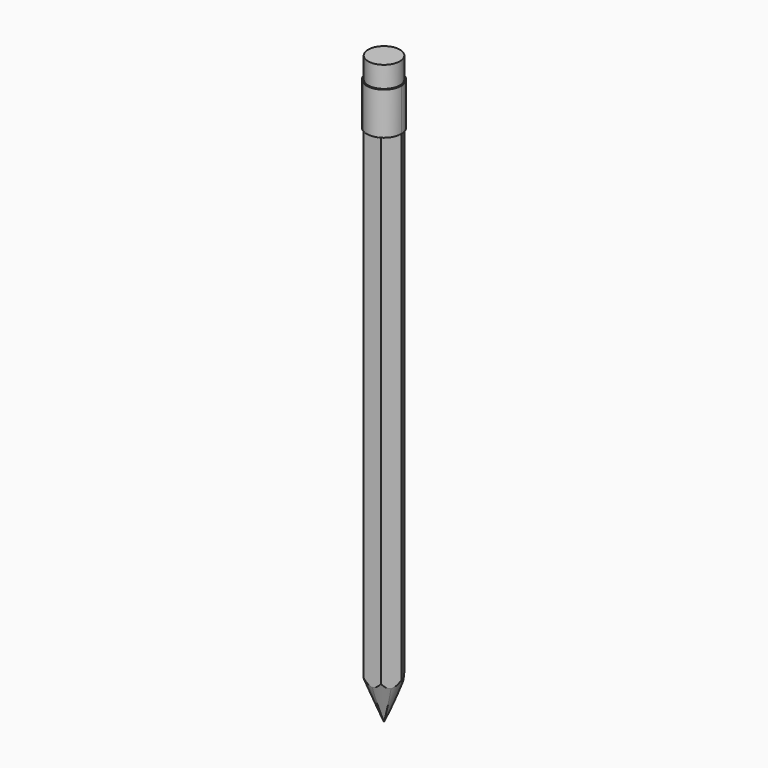
from build123d import *

# Parameters (mm, degrees)
F1_DEPTH     = 2540
F3_DEPTH     = 203.2
F4_R         = 76.1921609871
F5_DEPTH     = 101.6
F6_SIZE2     = 203.2
F6_SIZE      = 71.882
F7_T1_DEPTH  = 494.4083201135
F7_T3_DEPTH  = 494.4083201135
F7_T5_DEPTH  = 494.4083201135
F7_T7_DEPTH  = 494.4083201135
F7_T9_DEPTH  = 494.4083201135
F7_T11_DEPTH = 494.4083201135


# Not quite as in the source:
# - a fillet or chamfer that OpenCascade refuses, or shapes differently, is made with other operations: its cross-section is extruded or revolved along the edge and cut away or added


with BuildPart() as f1:
    # F0 (on Top) → F1 (new body)
    with BuildSketch(Plane.XY):
        Polygon((42.1619373396, -71.5559341018), (83.0502253935, 0.735341758), (40.8882880539, 72.2912758598), (-42.1619373396, 71.5559341018), (-83.0502253935, -0.735341758), (-40.8882880539, -72.2912758598), align=None)
    extrude(amount=F1_DEPTH)

    # F2 (on face) → F3 (join)
    with BuildSketch(Plane.XY.offset(2540)):
        with BuildLine():
            ThreePointArc((-40.8882880539, -72.2912758598), (0.735341758, -83.0502253935), (42.1619373396, -71.5559341018))
            Line((42.1619373396, -71.5559341018), (-40.8882880539, -72.2912758598))
        make_face()
        with BuildLine():
            ThreePointArc((-83.0502253935, -0.735341758), (-71.5559341018, -42.1619373396), (-40.8882880539, -72.2912758598))
            Line((-40.8882880539, -72.2912758598), (-83.0502253935, -0.735341758))
        make_face()
        with BuildLine():
            Line((-83.0502253935, -0.735341758), (-42.1619373396, 71.5559341018))
            ThreePointArc((-42.1619373396, 71.5559341018), (-72.2912758598, 40.8882880539), (-83.0502253935, -0.735341758))
        make_face()
        Polygon((42.1619373396, -71.5559341018), (83.0502253935, 0.735341758), (40.8882880539, 72.2912758598), (-42.1619373396, 71.5559341018), (-83.0502253935, -0.735341758), (-40.8882880539, -72.2912758598), align=None)
        with BuildLine():
            ThreePointArc((42.1619373396, -71.5559341018), (72.1095566371, -41.2079180135), (83.0534807543, 0))
            ThreePointArc((83.0534807543, 0), (83.0526669101, 0.3676744818), (83.0502253935, 0.735341758))
            Line((83.0502253935, 0.735341758), (42.1619373396, -71.5559341018))
        make_face()
        with BuildLine():
            Line((40.8882880539, 72.2912758598), (83.0502253935, 0.735341758))
            ThreePointArc((83.0502253935, 0.735341758), (71.5559341018, 42.1619373396), (40.8882880539, 72.2912758598))
        make_face()
        with BuildLine():
            Line((-42.1619373396, 71.5559341018), (40.8882880539, 72.2912758598))
            ThreePointArc((40.8882880539, 72.2912758598), (-0.735341758, 83.0502253935), (-42.1619373396, 71.5559341018))
        make_face()
    extrude(amount=F3_DEPTH)

    # F4 (on face) → F5 (join)
    with BuildSketch(Plane.XY.offset(2743.2)):
        Circle(F4_R)
    extrude(amount=F5_DEPTH)

    # F6
    f6_edges = [f1.edges().sort_by_distance(p)[0] for p in [
        (62.606081, -35.410296, 0),
        (61.969257, 36.513309, 0),
        (-0.636825, 71.923605, 0),
        (-62.606081, 35.410296, 0),
        (-61.969257, -36.513309, 0),
        (0.636825, -71.923605, 0),
    ]]
    f6_side = f1.faces().sort_by_distance((0, 0, 0))[0]
    chamfer(f6_edges, length=F6_SIZE, length2=F6_SIZE2, reference=f6_side)

    # F7: fillet of radius 76.2 on 6 edges, made by hand

    # F7_s2 → F7_t1 (cut)
    with BuildSketch(Plane(origin=(-18.9514614698, -33.5065465998, -94.2401135792), x_dir=(-0.8704183762, 0.4923127566, 0), z_dir=(0.1861654151, 0.329144017, 0.9257465389))):
        with BuildLine():
            ThreePointArc((-35.9188045712, 19.1503954496), (0, 10.1536652969), (35.9188045712, 19.1503954496))
            Line((35.9188045712, 19.1503954496), (0, -0.0474877004))
            Line((0, -0.0474877004), (-35.9188045712, 19.1503954496))
        make_face()
    extrude(amount=F7_T1_DEPTH, mode=Mode.SUBTRACT)

    # F7_s4 → F7_t3 (cut)
    with BuildSketch(Plane(origin=(19.5417898136, -33.1657203716, -94.2401135792), x_dir=(-0.8615645419, -0.5076480475, 0), z_dir=(-0.1919643727, 0.3257959873, 0.9257465389))):
        with BuildLine():
            ThreePointArc((-35.9188045712, 19.1503954496), (0, 10.1536652969), (35.9188045712, 19.1503954496))
            Line((35.9188045712, 19.1503954496), (0, -0.0474877004))
            Line((0, -0.0474877004), (-35.9188045712, 19.1503954496))
        make_face()
    extrude(amount=F7_T3_DEPTH, mode=Mode.SUBTRACT)

    # F7_s6 → F7_t5 (cut)
    with BuildSketch(Plane(origin=(38.4932512834, 0.3408262282, -94.2401135792), x_dir=(0.0088538343, -0.999960804, 0), z_dir=(-0.3781297878, -0.0033480297, 0.9257465389))):
        with BuildLine():
            ThreePointArc((35.9188045712, 19.1503954496), (0, 10.1536652969), (-35.9188045712, 19.1503954496))
            Line((-35.9188045712, 19.1503954496), (0, -0.0474877004))
            Line((0, -0.0474877004), (35.9188045712, 19.1503954496))
        make_face()
    extrude(amount=F7_T5_DEPTH, mode=Mode.SUBTRACT)

    # F7_s8 → F7_t7 (cut)
    with BuildSketch(Plane(origin=(18.9514614698, 33.5065465998, -94.2401135792), x_dir=(0.8704183762, -0.4923127566, 0), z_dir=(-0.1861654151, -0.329144017, 0.9257465389))):
        with BuildLine():
            ThreePointArc((35.9188045712, 19.1503954496), (0, 10.1536652969), (-35.9188045712, 19.1503954496))
            Line((-35.9188045712, 19.1503954496), (0, -0.0474877004))
            Line((0, -0.0474877004), (35.9188045712, 19.1503954496))
        make_face()
    extrude(amount=F7_T7_DEPTH, mode=Mode.SUBTRACT)

    # F7_s10 → F7_t9 (cut)
    with BuildSketch(Plane(origin=(-19.5417898136, 33.1657203716, -94.2401135792), x_dir=(0.8615645419, 0.5076480475, 0), z_dir=(0.1919643727, -0.3257959873, 0.9257465389))):
        with BuildLine():
            ThreePointArc((35.9188045712, 19.1503954496), (0, 10.1536652969), (-35.9188045712, 19.1503954496))
            Line((-35.9188045712, 19.1503954496), (0, -0.0474877004))
            Line((0, -0.0474877004), (35.9188045712, 19.1503954496))
        make_face()
    extrude(amount=F7_T9_DEPTH, mode=Mode.SUBTRACT)

    # F7_s12 → F7_t11 (cut)
    with BuildSketch(Plane(origin=(-38.4932512834, -0.3408262282, -94.2401135792), x_dir=(-0.0088538343, 0.999960804, 0), z_dir=(0.3781297878, 0.0033480297, 0.9257465389))):
        with BuildLine():
            ThreePointArc((-35.9188045712, 19.1503954496), (0, 10.1536652969), (35.9188045712, 19.1503954496))
            Line((35.9188045712, 19.1503954496), (0, -0.0474877004))
            Line((0, -0.0474877004), (-35.9188045712, 19.1503954496))
        make_face()
    extrude(amount=F7_T11_DEPTH, mode=Mode.SUBTRACT)


solid = f1.part
